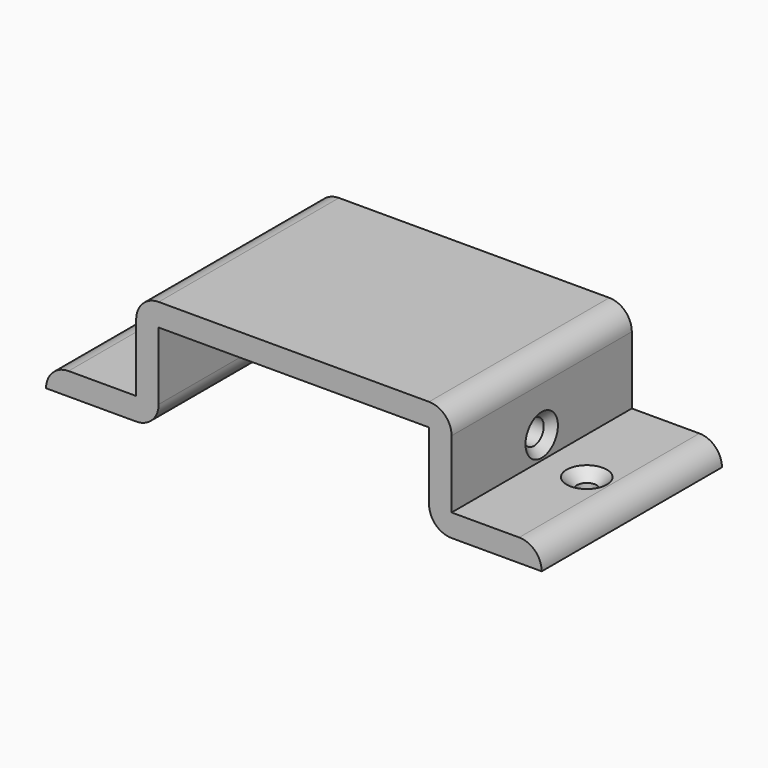
from build123d import *

# Parameters (mm, degrees)
F1_DEPTH             = 50
F4_D                 = 4.4
F4_CSINK_D           = 8.96
F4_CSINK_ANGLE       = 90
F4_ON_F3_D           = 4.4
F4_ON_F3_CSINK_D     = 8.96
F4_ON_F3_CSINK_ANGLE = 90
F6_D                 = 5.5
F6_DEPTH             = 5
F6_CSINK_D           = 9
F6_CSINK_ANGLE       = 90
F6_TIP               = 1.6523667023
F8_D                 = 5.5
F8_DEPTH             = 5
F8_CSINK_D           = 9
F8_CSINK_ANGLE       = 90
F8_TIP               = 1.6523667023
F9_R                 = 4.99999


# Not quite as in the source:
# - a fillet or chamfer is up to 0.001 mm smaller than in the source, because OpenCascade refuses the exact size


with BuildPart() as f1:
    # F0 (on Front) → F1 (new body)
    with BuildSketch(Plane.XZ):
        Polygon((-55, 5), (-55, 0), (-30, 0), (-30, 20), (30, 20), (30, 0), (55, 0), (55, 5), (35, 5), (35, 25), (-35, 25), (-35, 5), align=None)
    extrude(amount=F1_DEPTH)

    # F4 (through all)
    with Locations(Plane.XY.offset(5)):
        with Locations((-45, -25)):
            CounterSinkHole(F4_D / 2, F4_CSINK_D / 2, counter_sink_angle=F4_CSINK_ANGLE)

    # F4 on F3 (through all)
    with Locations(Plane.XY.offset(5)):
        with Locations((45, -25)):
            CounterSinkHole(F4_ON_F3_D / 2, F4_ON_F3_CSINK_D / 2, counter_sink_angle=F4_ON_F3_CSINK_ANGLE)

    # F6
    with Locations(Plane(origin=(-35, 0, 0), x_dir=(0, -1, 0), z_dir=(-1, 0, 0))):
        with Locations((25, 10)):
            CounterSinkHole(F6_D / 2, F6_CSINK_D / 2, depth=F6_DEPTH, counter_sink_angle=F6_CSINK_ANGLE)
            with Locations((0, 0, -(F6_DEPTH + F6_TIP / 2))):  # 118° drill point
                Cone(0, F6_D / 2, F6_TIP, mode=Mode.SUBTRACT)

    # F8
    with Locations(Plane.YZ.offset(35)):
        with Locations((-25, 10)):
            CounterSinkHole(F8_D / 2, F8_CSINK_D / 2, depth=F8_DEPTH, counter_sink_angle=F8_CSINK_ANGLE)
            with Locations((0, 0, -(F8_DEPTH + F8_TIP / 2))):  # 118° drill point
                Cone(0, F8_D / 2, F8_TIP, mode=Mode.SUBTRACT)

    # F9 (radius 5 in the source; OpenCascade refuses exactly that, so slightly less here)
    f9_edges = [f1.edges().sort_by_distance(p)[0] for p in [
        (-30, -25, 0),
        (30, -25, 0),
        (-55, -25, 5),
        (55, -25, 5),
        (-35, -25, 25),
        (35, -25, 25),
    ]]
    fillet(f9_edges, radius=F9_R)


solid = f1.part
